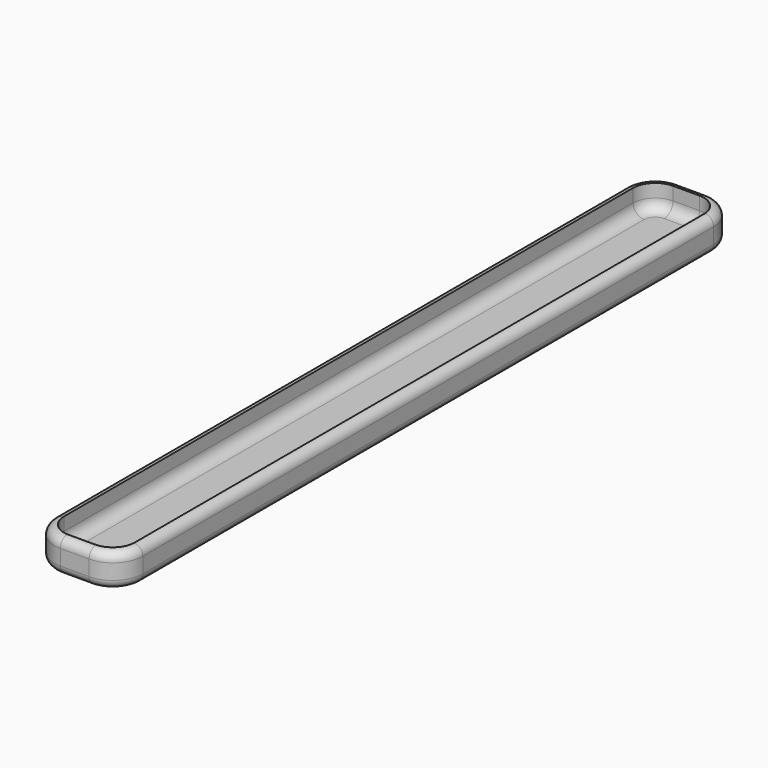
from build123d import *

# Parameters (mm, degrees)
F0_W     = 8
F0_H     = 70
F1_DEPTH = 3
F2_W     = 6.4
F2_H     = 68.4
F3_DEPTH = 2.2
F4_R     = 2.7
F5_R     = 2
F6_R     = 0.79999
F7_R     = 1


# Not quite as in the source:
# - a fillet or chamfer is up to 0.001 mm smaller than in the source, because OpenCascade refuses the exact size


with BuildPart() as f1:
    # F0 (on Top) → F1 (new body)
    with BuildSketch(Plane.XY):
        Rectangle(F0_W, F0_H)
    extrude(amount=F1_DEPTH)

    # F2 (on face) → F3 (cut)
    with BuildSketch(Plane.XY.offset(3)):
        Rectangle(F2_W, F2_H)
    extrude(amount=-F3_DEPTH, mode=Mode.SUBTRACT)

    # F4
    f4_edges = [f1.edges().sort_by_distance(p)[0] for p in [
        (4, -35, 1.5),
        (-4, -35, 1.5),
        (-4, 35, 1.5),
        (4, 35, 1.5),
    ]]
    fillet(f4_edges, radius=F4_R)

    # F5
    f5_edges = [f1.edges().sort_by_distance(p)[0] for p in [
        (-3.2, 34.2, 1.9),
        (3.2, 34.2, 1.9),
        (-3.2, -34.2, 1.9),
        (3.2, -34.2, 1.9),
    ]]
    fillet(f5_edges, radius=F5_R)

    # F6 (radius 0.8 in the source; OpenCascade refuses exactly that, so slightly less here)
    f6_edges = [f1.edges().sort_by_distance(p)[0] for p in [
        (-3.209188, -34.209188, 0),
        (-3.209188, -34.209188, 3),
    ]]
    fillet(f6_edges, radius=F6_R)

    # F7
    f7_edges = [f1.edges().sort_by_distance(p)[0] for p in [
        (-2.614214, -33.614214, 0.8),
    ]]
    fillet(f7_edges, radius=F7_R)


solid = f1.part
